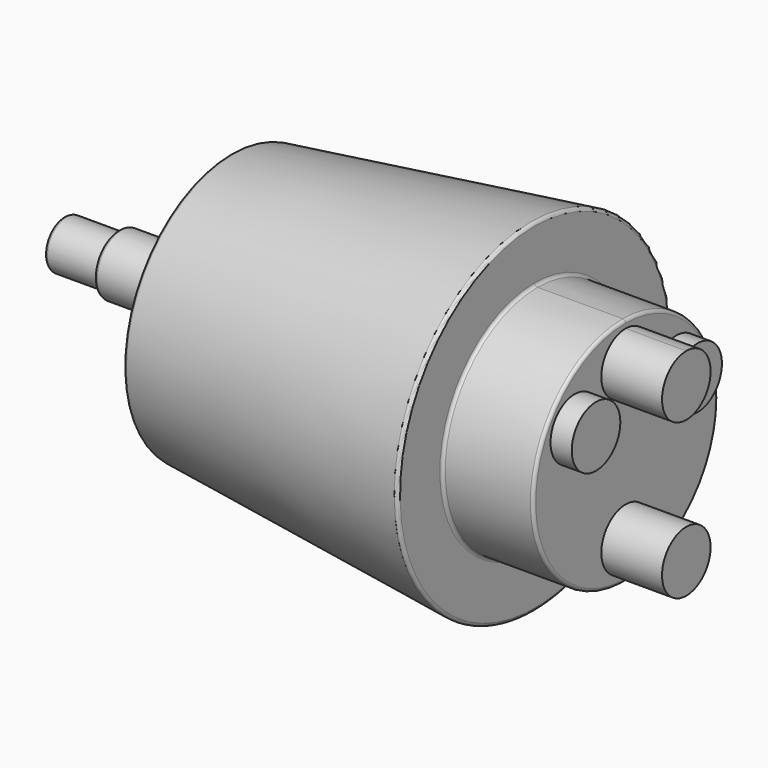
from build123d import *

# Parameters (mm, degrees)
F0_W     = 18
F0_H     = 8
F2_R     = 10
F3_DEPTH = 37
F4_DEPTH = 50
F5_DEPTH = 30
F6_R     = 1
F7_R     = 1


with BuildPart() as f1:
    # F0 (on Front) → F1 (revolve)
    with BuildSketch(Plane.XZ):
        with Locations((-105.3805270673, 4)):
            Rectangle(F0_W, F0_H)
        Polygon((-96.3805270673, 8), (-96.3805270673, 0), (-59.3805270673, 0), (-59.3805270673, 10), (-96.3805270673, 10), align=None)
        Polygon((-59.3805270673, 10), (-59.3805270673, 0), (40.6194729327, 0), (40.6194729327, 56.5), (-59.3805270673, 44), align=None)
    revolve(axis=Axis((8.274338072, 0, 0), (-1, 0, 0)))

    # F2 (on face) → F3 (join)
    with BuildSketch(Plane.YZ.offset(40.6194729327)):
        with Locations((-20.9141805002, 15)):
            Circle(F2_R)
        with Locations((20.9141805002, 15)):
            Circle(F2_R)
    extrude(amount=F3_DEPTH)

    # F2 (on face) → F4 (join)
    with BuildSketch(Plane.YZ.offset(40.6194729327)):
        with BuildLine():
            ThreePointArc((10, 25.5), (7.0710678119, 32.5710678119), (0, 35.5))
            ThreePointArc((0, 35.5), (-7.0710678119, 18.4289321881), (10, 25.5))
        make_face()
        with Locations((0, -25.5)):
            Circle(F2_R)
    extrude(amount=F4_DEPTH)

    # F2 (on face) → F5 (join)
    with BuildSketch(Plane.YZ.offset(40.6194729327)):
        with BuildLine():
            ThreePointArc((0, 38), (-26.8700576851, -26.8700576851), (38, 0))
            ThreePointArc((38, 0), (37.2205511714, 7.6570601732), (34.9141805002, 15))
            ThreePointArc((34.9141805002, 15), (20.9045449604, 31.7332633052), (0, 38))
        make_face()
        with Locations((0, -25.5)):
            Circle(F2_R, mode=Mode.SUBTRACT)
        with Locations((-20.9141805002, 15)):
            Circle(F2_R, mode=Mode.SUBTRACT)
        with BuildLine():
            ThreePointArc((10, 25.5), (-7.0710678119, 18.4289321881), (0, 35.5))
            ThreePointArc((0, 35.5), (7.0710678119, 32.5710678119), (10, 25.5))
        make_face(mode=Mode.SUBTRACT)
        with Locations((20.9141805002, 15)):
            Circle(F2_R, mode=Mode.SUBTRACT)
    extrude(amount=F5_DEPTH)

    # F6
    f6_edges = [f1.edges().sort_by_distance(p)[0] for p in [
        (-59.380527, 0, -44),
        (40.619473, 0, -56.5),
        (-96.380527, 0, -10),
        (-114.380527, 0, -8),
        (70.619473, -38, 0),
    ]]
    fillet(f6_edges, radius=F6_R)

    # F7
    f7_edges = [f1.edges().sort_by_distance(p)[0] for p in [
        (40.619473, -38, 0),
        (-59.380527, 0, -43.117218),
        (-59.380527, 0, -10),
    ]]
    fillet(f7_edges, radius=F7_R)


solid = f1.part
